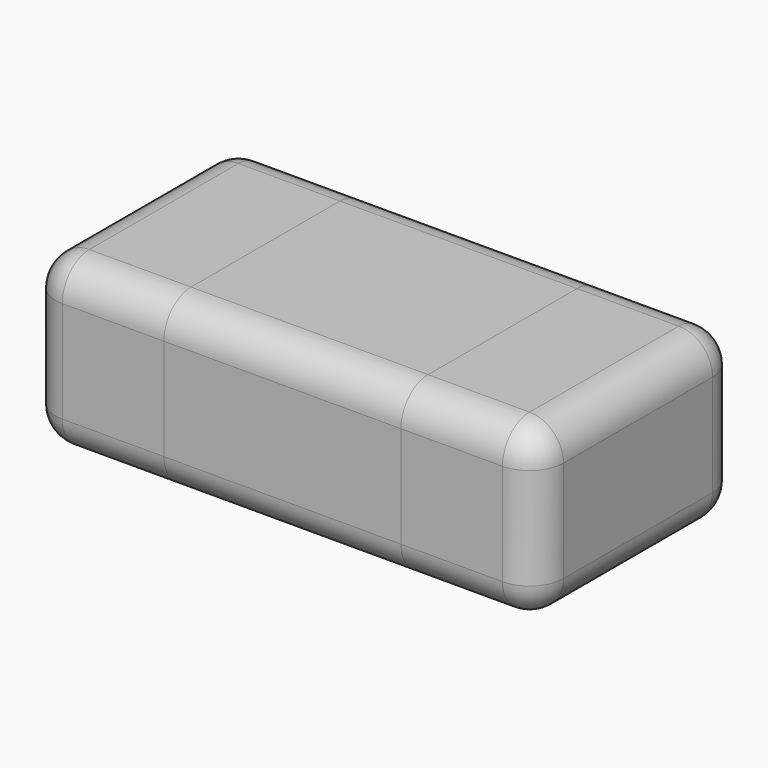
from build123d import *

# Parameters (mm, degrees)
F2_W     = 0.14
F2_H     = 0.15
F3_DEPTH = 0.08
F2_W_2   = 0.08
F4_DEPTH = 0.1
F5_DEPTH = 0.1
F6_DEPTH = 0.02
F7_R     = 0.01999
F7_2_R   = 0.01999
F7_3_R   = 0.01999
F7_4_R   = 0.01999


# Not quite as in the source:
# - a fillet or chamfer is up to 0.001 mm smaller than in the source, because OpenCascade refuses the exact size


with BuildPart() as f3:
    # F2 (on Top) → F3 (new body)
    with BuildSketch(Plane.XY):
        Rectangle(F2_W, F2_H)
    extrude(amount=F3_DEPTH)


with BuildPart() as f4:
    # F2 (on Top) → F4 (new body)
    with BuildSketch(Plane.XY):
        with Locations((-0.11, 0)):
            Rectangle(F2_W_2, F2_H)
    extrude(amount=F4_DEPTH)

    # F7 (radius 0.02 in the source; OpenCascade refuses exactly that, so slightly less here)
    f7_edges = [f4.edges().sort_by_distance(p)[0] for p in [
        (-0.11, -0.075, 0.1),
        (-0.15, 0.075, 0.05),
        (-0.15, -0.075, 0.05),
        (-0.15, 0, 0),
        (-0.15, 0, 0.1),
        (-0.11, 0.075, 0.1),
        (-0.11, 0.075, 0),
        (-0.11, -0.075, 0),
    ]]
    fillet(f7_edges, radius=F7_R)


with BuildPart() as f5:
    # F2 (on Top) → F5 (new body)
    with BuildSketch(Plane.XY):
        with Locations((0.11, 0)):
            Rectangle(F2_W_2, F2_H)
    extrude(amount=F5_DEPTH)

    # F7#2 (radius 0.02 in the source; OpenCascade refuses exactly that, so slightly less here)
    f7_2_edges = [f5.edges().sort_by_distance(p)[0] for p in [
        (0.11, -0.075, 0.1),
        (0.15, -0.075, 0.05),
        (0.15, 0.075, 0.05),
        (0.15, 0, 0),
        (0.15, 0, 0.1),
        (0.11, 0.075, 0.1),
        (0.11, 0.075, 0),
        (0.11, -0.075, 0),
    ]]
    fillet(f7_2_edges, radius=F7_2_R)


with BuildPart() as f6:
    # F6 (new): a face of the model
    f6_faces = [f3.part.faces().sort_by_distance(p)[0] for p in [
        (0, 0, 0.08),
    ]]
    extrude(f6_faces, amount=F6_DEPTH)

    # F7#4 (radius 0.02 in the source; OpenCascade refuses exactly that, so slightly less here)
    f7_4_edges = [f6.edges().sort_by_distance(p)[0] for p in [
        (0, -0.075, 0.1),
        (0, 0.075, 0.1),
    ]]
    fillet(f7_4_edges, radius=F7_4_R)


with BuildPart() as f3_1:
    add(f3.part)

    # F7#3 (radius 0.02 in the source; OpenCascade refuses exactly that, so slightly less here)
    f7_3_edges = [f3_1.edges().sort_by_distance(p)[0] for p in [
        (0, 0.075, 0),
        (0, -0.075, 0),
    ]]
    fillet(f7_3_edges, radius=F7_3_R)


solid = Compound([f4.part, f5.part, f6.part, f3_1.part])
